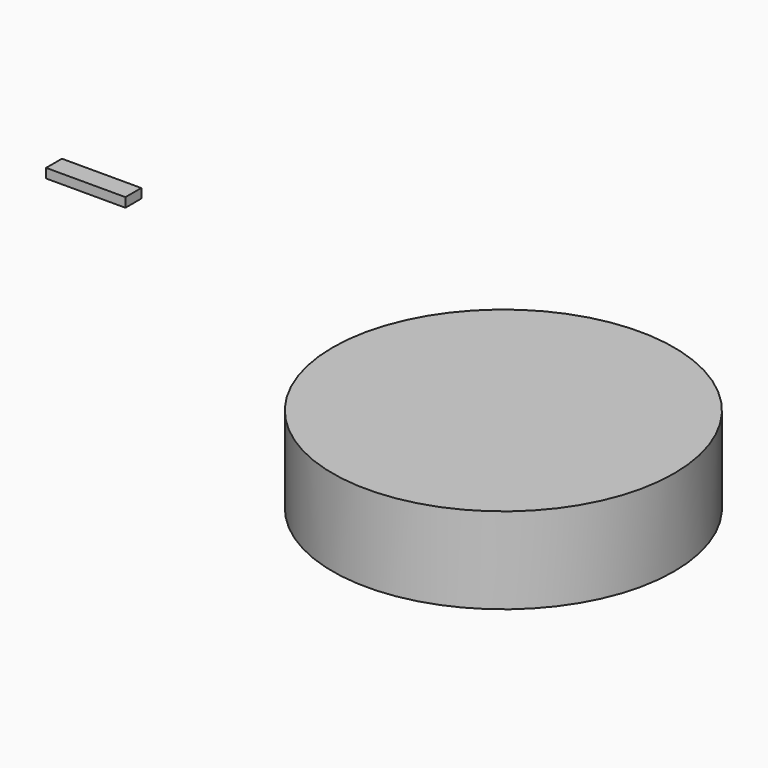
from build123d import *

# Parameters (mm, degrees)
F3_W     = 63.0901316181
F3_H     = 7.4481330812
F4_DEPTH = 7.874
F8_DEPTH = 68.58


# Not quite as in the source:
# - the program builds the solid bodies; features that only make, move or delete a surface that nothing else refers to are left out


with BuildPart() as f4:
    # F3 (on Front) → F4 (new body, symmetric)
    with BuildSketch(Plane.XZ):
        with Locations((-40.032423567, 53.3972028643)):
            Rectangle(F3_W, F3_H)
    extrude(amount=F4_DEPTH, both=True)


with BuildPart() as f8:
    # F7 (on Top) → F8 (new body)
    with BuildSketch(Plane.XY):
        with BuildLine():
            ThreePointArc((149.7005671263, 0.4245620221), (285.452902317, -135.3277731687), (421.2052375078, 0.4245620221))
            ThreePointArc((421.2052375078, 0.4245620221), (285.452902317, 136.1768972129), (149.7005671263, 0.4245620221))
        make_face()
    extrude(amount=-F8_DEPTH)


solid = Compound([f4.part, f8.part])
